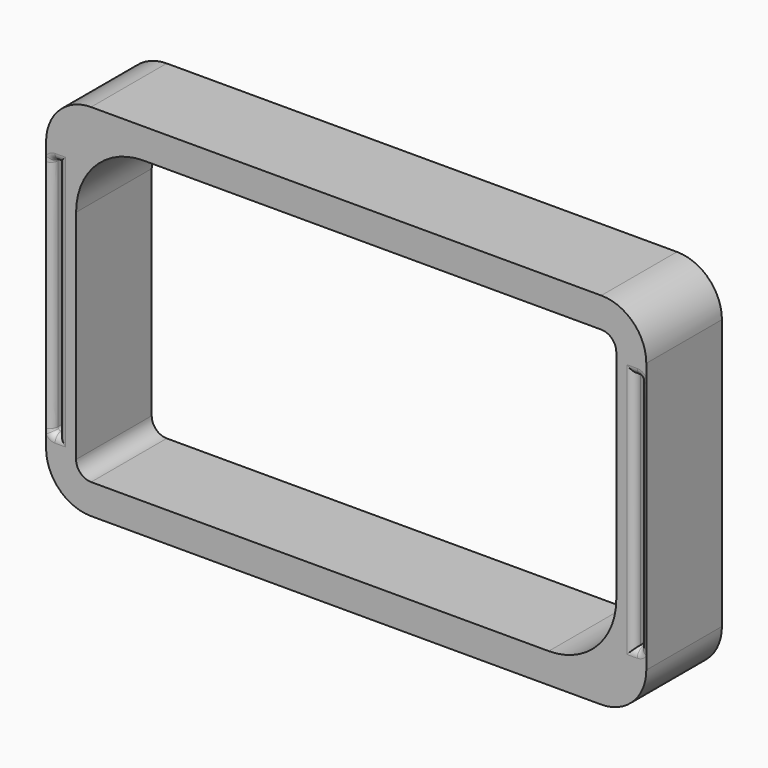
from build123d import *

# Parameters (mm, degrees)
F0_W     = 0.8
F0_H     = 32
F1_DEPTH = 6.3
F3_R     = 2.5
F4_DEPTH = 11
F5_R     = 2
F6_F1_R  = 0.4
F6_F2_R  = 0.4
F7_R     = 1


# Not quite as in the source:
# - a feature names something its author has since deleted; it is built from what else it names


with BuildPart() as f1:
    # F0 (on Front) → F1 (new body, symmetric)
    with BuildSketch(Plane.XZ):
        with BuildLine():
            Line((34, 24), (-34, 24))
            ThreePointArc((-34, 24), (-38.2426406871, 22.2426406871), (-40, 18))
            Line((-40, 18), (-40, -18))
            ThreePointArc((-40, -18), (-38.2426406871, -22.2426406871), (-34, -24))
            Line((-34, -24), (34, -24))
            ThreePointArc((34, -24), (38.2426406871, -22.2426406871), (40, -18))
            Line((40, -18), (40, 18))
            ThreePointArc((40, 18), (38.2426406871, 22.2426406871), (34, 24))
        make_face()
        with Locations((-38.8, 0)):
            Rectangle(F0_W, F0_H, mode=Mode.SUBTRACT)
        with BuildLine():
            ThreePointArc((-36, 11), (-33.3639610307, 17.3639610307), (-27, 20))
            Line((-27, 20), (34, 20))
            ThreePointArc((34, 20), (35.4142135624, 19.4142135624), (36, 18))
            Line((36, 18), (36, -11))
            ThreePointArc((36, -11), (33.3639610307, -17.3639610307), (27, -20))
            Line((27, -20), (-34, -20))
            ThreePointArc((-34, -20), (-35.4142135624, -19.4142135624), (-36, -18))
            Line((-36, -18), (-36, 11))
        make_face(mode=Mode.SUBTRACT)
        with Locations((38.8, 0)):
            Rectangle(F0_W, F0_H, mode=Mode.SUBTRACT)
    extrude(amount=F1_DEPTH, both=True)

    # F3 (on offset) → F4 (cut)
    with BuildSketch(Plane.XZ.offset(5.5)):
        with Locations((-34.9874263129, 20.2)):
            Circle(F3_R)
        with Locations((34.9874263129, -20.2)):
            Circle(F3_R)
    extrude(amount=-F4_DEPTH, mode=Mode.SUBTRACT)

    # F5
    f5_edges = [f1.edges().sort_by_distance(p)[0] for p in [
        (-38.4, 6.3, 0),
        (38.4, 6.3, 0),
    ]]
    fillet(f5_edges, radius=F5_R)

    # F6: fillet of radius 0.4 on 8 edges, made by hand

    # F6_f1
    f6_f1_edges = [f1.edges().sort_by_distance(p)[0] for p in [
        (-39.2, 0, 16),
        (-39.2, 0, -16),
        (39.2, 0, -16),
        (39.2, 0, 16),
    ]]
    fillet(f6_f1_edges, radius=F6_F1_R)

    # F6_f2
    f6_f2_edges = [f1.edges().sort_by_distance(p)[0] for p in [
        (38.6, 6.3, 16),
        (-38.6, 6.3, 16),
        (-39.2, 6.3, 0),
        (39.2, 6.3, 0),
        (-37.4, 6.3, 16),
        (37.4, 6.3, 16),
        (39.0828427125, 6.3, 15.8828427125),
        (39.0828427125, 6.3, -15.8828427125),
        (-39.0828427125, 6.3, -15.8828427125),
        (-39.0828427125, 6.3, 15.8828427125),
    ]]
    fillet(f6_f2_edges, radius=F6_F2_R)

    # F7
    f7_edges = [f1.edges().sort_by_distance(p)[0] for p in [
        (38.4, -6.3, 0),
        (39.2, -6.3, 0),
        (-38.4, -6.3, 0),
        (-39.2, -6.3, 0),
        (38.6, -6.3, -16),
        (38.6, -6.3, 16),
        (-38.6, -6.3, -16),
        (-38.6, -6.3, 16),
    ]]
    fillet(f7_edges, radius=F7_R)


solid = f1.part
